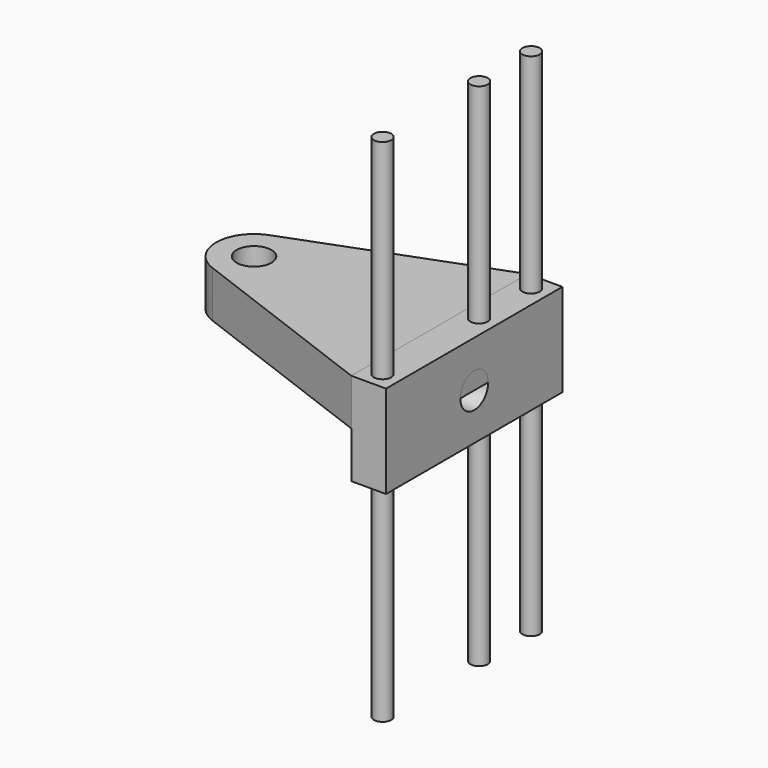
from build123d import *

# Parameters (mm, degrees)
F0_R     = 4.7625
F1_DEPTH = 139.7
F0_W     = 19.05
F0_H     = 120.65
F0_R_2   = 9.525
F2_DEPTH = 25.4
F3_DEPTH = 25.4
F4_R     = 22.225
F4_R_2   = 9.525
F5_DEPTH = 88.9
F6_DEPTH = 141.2596404097


with BuildPart() as f1:
    # F0 (on Top) → F1 (new body, symmetric)
    with BuildSketch(Plane.XY):
        with Locations((111.0077798367, 50.8)):
            Circle(F0_R)
    extrude(amount=F1_DEPTH, both=True)


with BuildPart() as f1b:
    # F0 (on Top) → F1, piece 2 (new body, symmetric)
    with BuildSketch(Plane.XY):
        with Locations((111.0077798367, 15.24)):
            Circle(F0_R)
    extrude(amount=F1_DEPTH, both=True)


with BuildPart() as f1c:
    # F0 (on Top) → F1, piece 3 (new body, symmetric)
    with BuildSketch(Plane.XY):
        with Locations((111.0077798367, -50.8)):
            Circle(F0_R)
    extrude(amount=F1_DEPTH, both=True)


with BuildPart() as f2:
    # F0 (on Top) → F2 (new body)
    with BuildSketch(Plane.XY):
        with Locations((111.0077798367, 0)):
            Rectangle(F0_W, F0_H)
        with Locations((111.0077798367, -50.8)):
            Circle(F0_R, mode=Mode.SUBTRACT)
        with Locations((111.0077798367, 15.24)):
            Circle(F0_R, mode=Mode.SUBTRACT)
        with Locations((111.0077798367, 50.8)):
            Circle(F0_R, mode=Mode.SUBTRACT)
        with BuildLine():
            Line((101.4827798367, -60.325), (101.4827798367, 60.325))
            Line((101.4827798367, 60.325), (-7.298240398, 19.3983757977))
            ThreePointArc((-7.298240398, 19.3983757977), (-20.7258605731, 0), (-7.298240398, -19.3983757977))
            Line((-7.298240398, -19.3983757977), (101.4827798367, -60.325))
        make_face()
        Circle(F0_R_2, mode=Mode.SUBTRACT)
    extrude(amount=F2_DEPTH)


with BuildPart() as f3:
    # F0 (on Top) → F3 (new body, symmetric)
    with BuildSketch(Plane.XY):
        with Locations((111.0077798367, 0)):
            Rectangle(F0_W, F0_H)
        with Locations((111.0077798367, -50.8)):
            Circle(F0_R, mode=Mode.SUBTRACT)
        with Locations((111.0077798367, 15.24)):
            Circle(F0_R, mode=Mode.SUBTRACT)
        with Locations((111.0077798367, 50.8)):
            Circle(F0_R, mode=Mode.SUBTRACT)
    extrude(amount=F3_DEPTH, both=True)

    # F4 (on face) → F5 (join)
    with BuildSketch(Plane.YZ.offset(120.5327798367)):
        Circle(F4_R)
        Circle(F4_R_2, mode=Mode.SUBTRACT)
    extrude(amount=-F5_DEPTH)

    # F4 (on face) → F6 (cut, through all)
    with BuildSketch(Plane.YZ.offset(120.5327798367)):
        Circle(F4_R_2)
    extrude(amount=-F6_DEPTH, mode=Mode.SUBTRACT)


solid = Compound([f1.part, f1b.part, f1c.part, f2.part, f3.part])
